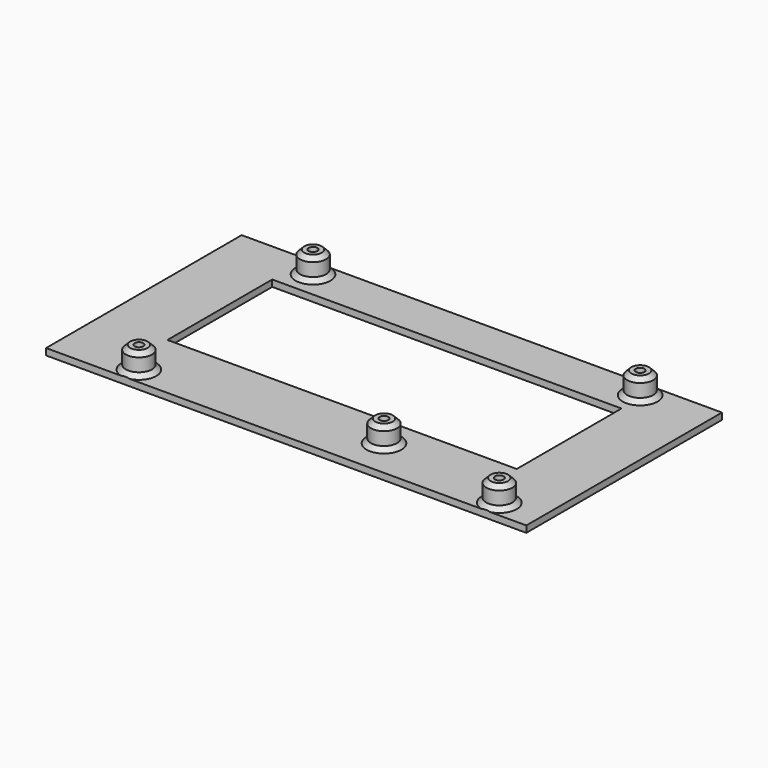
from build123d import *

# Parameters (mm, degrees)
F0_W     = 110
F0_H     = 56
F0_W_2   = 80
F0_H_2   = 30
F1_DEPTH = 1.5
F2_R     = 3
F2_R_2   = 1
F3_DEPTH = 5


# Not quite as in the source:
# - a fillet or chamfer that OpenCascade refuses, or shapes differently, is made with other operations: its cross-section is extruded or revolved along the edge and cut away or added


with BuildPart() as f1:
    # F0 (on Top) → F1 (new body)
    with BuildSketch(Plane.XY):
        Rectangle(F0_W, F0_H)
        with Locations((0, 3)):
            Rectangle(F0_W_2, F0_H_2, mode=Mode.SUBTRACT)
    extrude(amount=F1_DEPTH)

    # F2 (on face) → F3 (join)
    with BuildSketch(Plane.XY.offset(1.5)):
        with Locations((-35.56, 24.13)):
            Circle(F2_R)
        with Locations((-35.56, 24.13)):
            Circle(F2_R_2, mode=Mode.SUBTRACT)
        with Locations((39.37, 24.13)):
            Circle(F2_R)
        with Locations((39.37, 24.13)):
            Circle(F2_R_2, mode=Mode.SUBTRACT)
        with Locations((-36.83, -24.13)):
            Circle(F2_R)
        with Locations((-36.83, -24.13)):
            Circle(F2_R_2, mode=Mode.SUBTRACT)
        with Locations((15.24, -19.05)):
            Circle(F2_R)
        with Locations((15.24, -19.05)):
            Circle(F2_R_2, mode=Mode.SUBTRACT)
        with Locations((45.72, -24.13)):
            Circle(F2_R)
        with Locations((45.72, -24.13)):
            Circle(F2_R_2, mode=Mode.SUBTRACT)
    extrude(amount=F3_DEPTH)

    # F4: chamfer of 1 on 10 edges, made by hand


with BuildPart() as f4_tool2:
    # F4_s3 → F4_t4 (revolve)
    with BuildSketch(Plane.XZ.offset(-24.13)):
        Polygon((-31.56, 1.5), (-32.56, 2.5), (-32.56, 1.5), align=None)
    revolve(axis=Axis((-35.56, 24.13, 1.5), (0, 0, 1)))

    split(bisect_by=Plane.XZ.offset(-28), keep=Keep.TOP)


with BuildPart() as f1_1:
    add(f1.part)

    # F4_t1: union F4_tool2
    add(f4_tool2.part)


with BuildPart() as f4_tool7:
    # F4_s8 → F4_t9 (revolve)
    with BuildSketch(Plane.XZ.offset(-24.13)):
        Polygon((43.37, 1.5), (42.37, 2.5), (42.37, 1.5), align=None)
    revolve(axis=Axis((39.37, 24.13, 1.5), (0, 0, 1)))

    split(bisect_by=Plane.XZ.offset(-28), keep=Keep.TOP)


with BuildPart() as f1_2:
    add(f1_1.part)

    # F4_t6: union F4_tool7
    add(f4_tool7.part)


with BuildPart() as f4_tool12:
    # F4_s13 → F4_t14 (revolve)
    with BuildSketch(Plane.XZ.offset(24.13)):
        Polygon((49.72, 1.5), (48.72, 2.5), (48.72, 1.5), align=None)
    revolve(axis=Axis((45.72, -24.13, 1.5), (0, 0, 1)))

    split(bisect_by=Plane.XZ.offset(28), keep=Keep.BOTTOM)


with BuildPart() as f1_3:
    add(f1_2.part)

    # F4_t11: union F4_tool12
    add(f4_tool12.part)

    # F4_s16 → F4_t17 (revolve)
    with BuildSketch(Plane.XZ.offset(19.05)):
        Polygon((19.24, 1.5), (18.24, 2.5), (18.24, 1.5), align=None)
    revolve(axis=Axis((15.24, -19.05, 1.5), (0, 0, 1)))


with BuildPart() as f4_tool19:
    # F4_s20 → F4_t21 (revolve)
    with BuildSketch(Plane.XZ.offset(24.13)):
        Polygon((-32.83, 1.5), (-33.83, 2.5), (-33.83, 1.5), align=None)
    revolve(axis=Axis((-36.83, -24.13, 1.5), (0, 0, 1)))

    split(bisect_by=Plane.XZ.offset(28), keep=Keep.BOTTOM)


with BuildPart() as f1_4:
    add(f1_3.part)

    # F4_t18: union F4_tool19
    add(f4_tool19.part)

    # F4_s23 → F4_t24 (revolve, cut)
    with BuildSketch(Plane.XZ.offset(24.13)):
        Polygon((-33.83, 5.5), (-34.83, 6.5), (-33.83, 6.5), align=None)
    revolve(axis=Axis((-36.83, -24.13, 6.5), (0, 0, 1)), mode=Mode.SUBTRACT)

    # F4_s25 → F4_t26 (revolve, cut)
    with BuildSketch(Plane.XZ.offset(-24.13)):
        Polygon((-32.56, 5.5), (-33.56, 6.5), (-32.56, 6.5), align=None)
    revolve(axis=Axis((-35.56, 24.13, 6.5), (0, 0, 1)), mode=Mode.SUBTRACT)

    # F4_s27 → F4_t28 (revolve, cut)
    with BuildSketch(Plane.XZ.offset(-24.13)):
        Polygon((42.37, 5.5), (41.37, 6.5), (42.37, 6.5), align=None)
    revolve(axis=Axis((39.37, 24.13, 6.5), (0, 0, 1)), mode=Mode.SUBTRACT)

    # F4_s29 → F4_t30 (revolve, cut)
    with BuildSketch(Plane.XZ.offset(24.13)):
        Polygon((48.72, 5.5), (47.72, 6.5), (48.72, 6.5), align=None)
    revolve(axis=Axis((45.72, -24.13, 6.5), (0, 0, 1)), mode=Mode.SUBTRACT)

    # F4_s31 → F4_t32 (revolve, cut)
    with BuildSketch(Plane.XZ.offset(19.05)):
        Polygon((18.24, 5.5), (17.24, 6.5), (18.24, 6.5), align=None)
    revolve(axis=Axis((15.24, -19.05, 6.5), (0, 0, 1)), mode=Mode.SUBTRACT)


solid = f1_4.part
